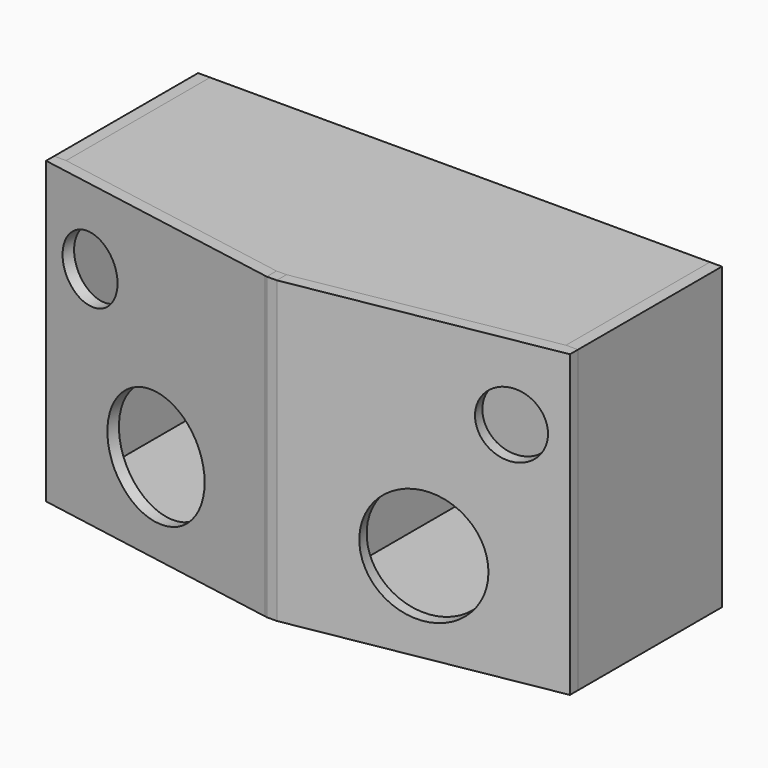
from build123d import *

# Parameters (mm, degrees)
F1_DEPTH  = 10
F2_DEPTH  = 300
F3_DEPTH  = 300
F4_W      = 180
F4_H      = 10
F4_H_2    = 290
F5_DEPTH  = 12
F6_W      = 180
F6_H      = 10
F6_H_2    = 290
F7_DEPTH  = 12
F8_W      = 12
F8_H      = 280
F9_DEPTH  = 500
F10_R     = 32.5
F10_R_2   = 57.5
F11_DEPTH = 25
F12_R     = 57.5
F12_R_2   = 32.5
F13_DEPTH = 25
F15_DEPTH = 10
F17_W     = 100
F17_H     = 10
F18_DEPTH = 245
F19_DEPTH = 255
F16_W     = 10
F16_H     = 60
F20_DEPTH = 245
F21_DEPTH = 255
F23_R     = 15
F24_DEPTH = 25


# Not quite as in the source:
# - a feature names something its author has since deleted; it is built from what else it names


with BuildPart() as f1:
    # F0 (on Top) → F1 (new body)
    with BuildSketch(Plane.XY):
        Polygon((500, 0), (0, 0), (0, -180), (245, -223.2001102736), (255, -223.2001102736), (500, -180), align=None)
    extrude(amount=F1_DEPTH)


with BuildPart() as f2:
    # F0 (on Top) → F2 (new body)
    with BuildSketch(Plane.XY):
        Polygon((245, -223.2001102736), (0, -180), (-12, -180), (-12, -190.0691955741), (242.916221868, -235.0178033097), (245, -235.3852296162), align=None)
    extrude(amount=F2_DEPTH)

    # F10 (on face) → F11 (cut)
    with BuildSketch(Plane(origin=(-32.8655910313, -186.3900289069, 0), x_dir=(0.984807753, -0.1736481777, 0), z_dir=(-0.1736481777, -0.984807753, 0))):
        with Locations((73.1874764059, 225)):
            Circle(F10_R)
        with Locations((151.1874764059, 90)):
            Circle(F10_R_2)
    extrude(amount=-F11_DEPTH, mode=Mode.SUBTRACT)


with BuildPart() as f3:
    # F0 (on Top) → F3 (new body)
    with BuildSketch(Plane.XY):
        Polygon((512, -180), (500, -180), (255, -223.2001102736), (255, -235.3852296162), (512, -190.0691955741), align=None)
    extrude(amount=F3_DEPTH)

    # F12 (on face) → F13 (cut)
    with BuildSketch(Plane(origin=(47.9424358348, -271.8950647383, 0), x_dir=(0.984807753, 0.1736481777, 0), z_dir=(0.1736481777, -0.984807753, 0))):
        with Locations((341.2164001002, 90)):
            Circle(F12_R)
        with Locations((419.2164001002, 225)):
            Circle(F12_R_2)
    extrude(amount=-F13_DEPTH, mode=Mode.SUBTRACT)


with BuildPart() as f5:
    # F4 (on face) → F5 (new body)
    with BuildSketch(Plane(origin=(0, 0, 0), x_dir=(0, -1, 0), z_dir=(-1, 0, 0))):
        with Locations((90, 5)):
            Rectangle(F4_W, F4_H)
        with Locations((90, 155)):
            Rectangle(F4_W, F4_H_2)
    extrude(amount=F5_DEPTH)


with BuildPart() as f7:
    # F6 (on face) → F7 (new body)
    with BuildSketch(Plane.YZ.offset(500)):
        with Locations((-90, 5)):
            Rectangle(F6_W, F6_H)
        with Locations((-90, 155)):
            Rectangle(F6_W, F6_H_2)
    extrude(amount=F7_DEPTH)


with BuildPart() as f9:
    # F8 (on face) → F9 (new body, through all)
    with BuildSketch(Plane.YZ):
        with Locations((-6, 150)):
            Rectangle(F8_W, F8_H)
    extrude(amount=F9_DEPTH)

    # F23 (on face) → F24 (cut)
    with BuildSketch(Plane(origin=(0, 0, 0), x_dir=(-1, 0, 0), z_dir=(0, 1, 0))):
        with Locations((-475, 265)):
            Circle(F23_R)
        with Locations((-25, 265)):
            Circle(F23_R)
    extrude(amount=-F24_DEPTH, mode=Mode.SUBTRACT)


with BuildPart() as f15:
    # F14 (on face) → F15 (new body)
    with BuildSketch(Plane.YZ.offset(245)):
        Polygon((-223.2001102736, 10), (-180, 10), (-12, 10), (-12, 230), (-122, 230), (-122, 290), (-223.2001102736, 290), align=None)
        Polygon((-223.2001102736, 0), (-223.2001102736, 10), (-223.2001102736, 290), (-223.2001102736, 300), (-235.3852296162, 300), (-235.3852296162, 0), align=None)
    extrude(amount=F15_DEPTH)


with BuildPart() as f18:
    # F17 (on face) → F18 (new body, through all)
    with BuildSketch(Plane.YZ.offset(255)):
        with Locations((-62, 235)):
            Rectangle(F17_W, F17_H)
    extrude(amount=F18_DEPTH)

    # F19 (add, through all): a face of the model
    f19_faces = [f18.faces().sort_by_distance(p)[0] for p in [
        (255, -62, 235),
    ]]
    extrude(f19_faces, amount=F19_DEPTH)


with BuildPart() as f20:
    # F16 (on face) → F20 (new body, through all)
    with BuildSketch(Plane.YZ.offset(255)):
        with Locations((-117, 260)):
            Rectangle(F16_W, F16_H)
    extrude(amount=F20_DEPTH)

    # F21 (add, through all): a face of the model
    f21_faces = [f20.faces().sort_by_distance(p)[0] for p in [
        (255, -117, 260),
    ]]
    extrude(f21_faces, amount=F21_DEPTH)


with BuildPart() as f22_1:
    # F22: copy of F1
    add(f1.part.moved(Location((0, 0, 290))))


solid = Compound([f1.part, f2.part, f3.part, f5.part, f7.part, f9.part, f15.part, f18.part, f20.part, f22_1.part])
